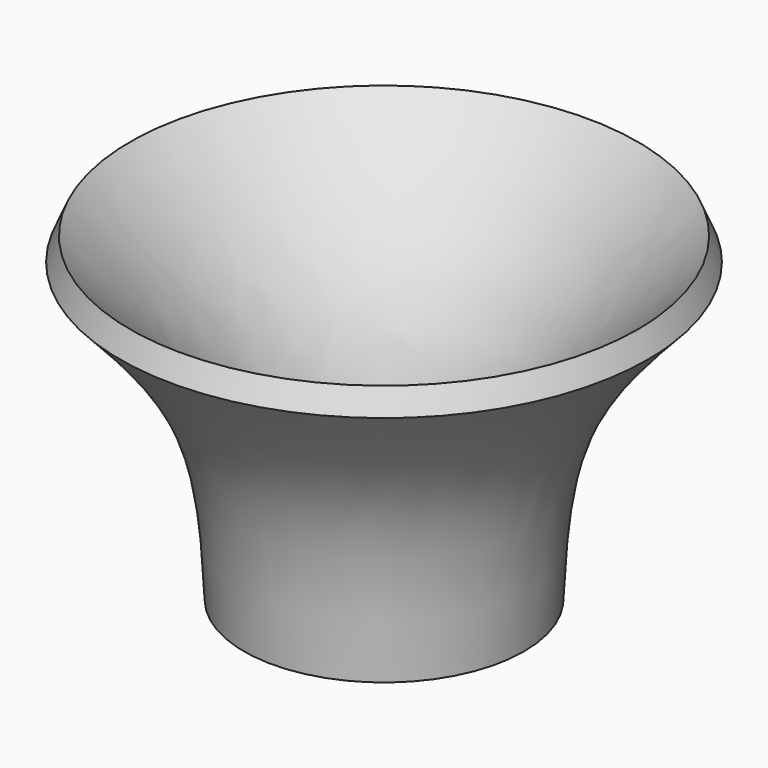
from build123d import *

# Parameters (mm, degrees)
F2_T = -2.54


# Not quite as in the source:
# - a fillet or chamfer that OpenCascade refuses, or shapes differently, is made with other operations: its cross-section is extruded or revolved along the edge and cut away or added


with BuildPart() as f1:
    # F0 (on Front) → F1 (revolve)
    with BuildSketch(Plane.XZ):
        with BuildLine():
            Line((0, 35.9757170081), (0, 0))
            Line((0, 0), (15.2537068352, 0))
            add(Edge.make_bspline(
                [(15.2537068352, 0), (15.555006608, 6.3278842639), (16.1857166232, 19.5740276097), (26.728109148, 30.3484172632), (32.2342403233, 35.9757170081)],
                knots=[0, 0, 0, 0, 0.4777152186, 1, 1, 1, 1], degree=3))
            Line((32.2342403233, 35.9757170081), (0, 35.9757170081))
        make_face()
    revolve(axis=Axis((0, 0, 17.9878585041), (0, 0, 1)))

    # F2
    f2_openings = [f1.faces().sort_by_distance(p)[0] for p in [
        (0, 0, 35.975717),
    ]]
    offset(amount=F2_T, openings=f2_openings)

    # F3: chamfer of 5.08 on 1 edges, made by hand

    # F3_s1 → F3_t2 (revolve, cut)
    with BuildSketch(Plane.XZ):
        with BuildLine():
            Line((28.8153241643, 32.1795455561), (27.1071352084, 36.1624665125))
            Line((27.1071352084, 36.1624665125), (27.1071352084, 36.2640665125))
            ThreePointArc((27.1071352084, 36.2640665125), (29.6706877658, 36.0773170081), (32.2342403233, 36.0773170081))
            Line((32.2342403233, 36.0773170081), (32.3068599509, 35.9046610464))
            ThreePointArc((32.3068599509, 35.9046610464), (30.524085875, 34.0783077951), (28.8889329129, 32.1095147619))
            Line((28.8889329129, 32.1095147619), (28.8153241643, 32.1795455561))
        make_face()
    revolve(axis=Axis((0, 0, 35.9757170081), (0, 0, 1)), mode=Mode.SUBTRACT)


solid = f1.part
